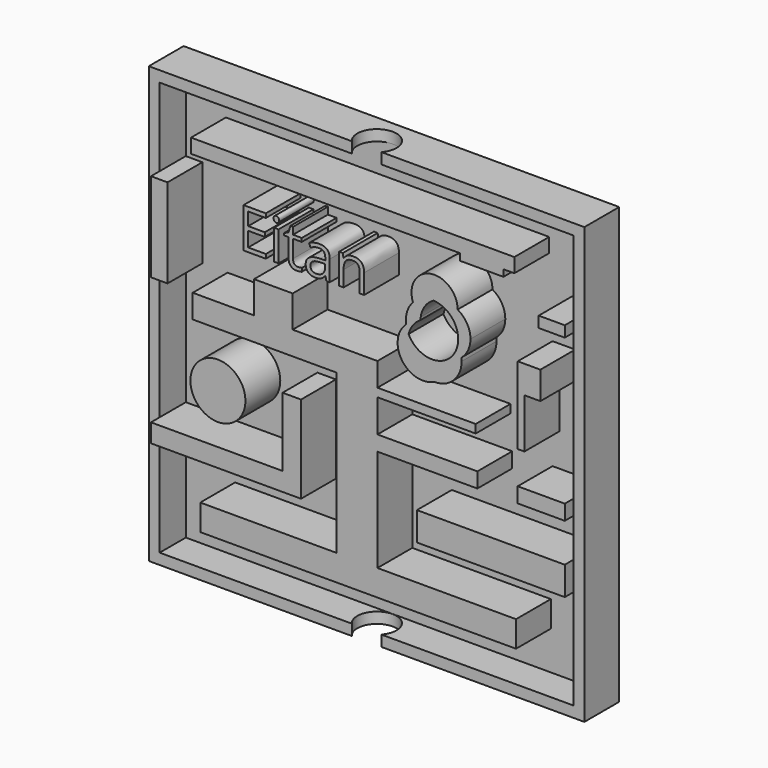
from build123d import *

# Parameters (mm, degrees)
F0_W         = 100
F0_H         = 100
F1_DEPTH     = 10
F2_T         = -2.5
F4_D         = 9
F5_W         = 22.9406361468
F5_H         = 3.4700129181
F5_W_2       = 22.5550816394
F5_H_2       = 1.9277847605
F5_W_3       = 8.8678086177
F5_H_3       = 7.3255812749
F5_W_4       = 4.2411256582
F5_H_4       = 15.8078335226
F5_R         = 6.314782536
F5_W_5       = 10.0244823843
F5_H_5       = 1.5422254801
F5_W_6       = 3.8039235713
F5_H_6       = 20.4345164821
F5_W_7       = 33.940872593
F5_H_7       = 6.5544676036
F5_W_8       = 10.8074559329
F5_W_9       = 1.5422254801
F5_H_8       = 17.7356194472
F5_W_10      = 5.9879957197
F5_H_9       = 2.5061201304
F5_TEXT_SIZE = 12.8518971097
F6_DEPTH     = 10
F7_W         = 3.6627911031
F7_H         = 6.3616903499
F8_DEPTH     = 10


# Not quite as in the source:
# - Text() gives the source's letters only with a copy of the font that has no kerning and outlines rounded to 1/6400 em; it was checked with that copy


with BuildPart() as f1:
    # F0 (on Front) → F1 (new body)
    with BuildSketch(Plane.XZ):
        with Locations((0.3209233341, -0.195864588)):
            Rectangle(F0_W, F0_H)
    extrude(amount=F1_DEPTH)

    # F2
    f2_openings = [f1.faces().sort_by_distance(p)[0] for p in [
        (0.320923, -10, -0.195865),
    ]]
    offset(amount=F2_T, openings=f2_openings)

    # F4 (through all)
    with Locations(Plane(origin=(0, 0, -50.195864588), x_dir=(1, 0, 0), z_dir=(0, 0, -1))):
        with Locations((0.3209233341, 7.0364135318)):
            Hole(F4_D / 2)

    # F5 (on face) → F6 (join)
    with BuildSketch(Plane.XZ.offset(2.5)):
        Polygon((-4.6266834252, -32.8687280416), (-35.8567945659, -32.8687280416), (-35.8567945659, -38.8448610902), (36.627907306, -38.8448610902), (36.627907306, -32.8687280416), (4.8194616102, -32.8687280416), align=None)
        Polygon((-4.6266834252, 0), (-4.6266834252, -32.8687280416), (4.8194616102, -32.8687280416), (4.8194616102, -10.5064269155), (4.8194616102, -9.3497559428), (4.8194616102, -5.8797430247), (4.8194616102, 0), align=None)
        Polygon((-4.6266834252, 3.5664017778), (-4.6266834252, 0), (4.8194616102, 0), (4.8194616102, 1.6386170173), (4.8194616102, 3.5664017778), align=None)
        Polygon((-4.8194616102, 3.5664017778), (-4.6266834252, 3.5664017778), (4.8194616102, 3.5664017778), (4.8194616102, 8.9641986415), (-4.8194616102, 8.9641986415), align=None)
        with Locations((16.2897796836, -7.6147494838)):
            Rectangle(F5_W, F5_H)
        with Locations((16.0970024299, 2.6025093975)):
            Rectangle(F5_W_2, F5_H_2)
        Polygon((-37.5918000937, 3.5664017778), (-4.8194616102, 3.5664017778), (-4.8194616102, 8.9641986415), (-14.6511634812, 8.9641986415), (-23.5189720988, 8.9641986415), (-37.5918000937, 8.9641986415), align=None)
        with Locations((-19.08506779, 12.6269892789)):
            Rectangle(F5_W_3, F5_H_3)
        Polygon((-47.1790766659, -20.3381273896), (-47.1790766659, -24.5792549103), (-12.7233788371, -24.5792549103), (-12.7233788371, -20.3381273896), (-16.9645044953, -20.3381273896), align=None)
        with Locations((-14.8439416662, -12.4342106283)):
            Rectangle(F5_W_4, F5_H_4)
        with Locations((-31.8084470928, -8.9641986415)):
            Circle(F5_R)
        Polygon((36.2423509359, 40.1943102479), (-37.9773564637, 40.1943102479), (-37.9773564637, 36.9170755148), (23.7117502838, 36.9170755148), (33.7362326682, 36.9170755148), (36.2423509359, 36.9170755148), align=None)
        with Locations((28.723991476, 36.1459627748)):
            Rectangle(F5_W_5, F5_H_5)
        with Locations((-45.2771148802, 19.1814568825)):
            Rectangle(F5_W_6, F5_H_6)
        with Locations((30.8504870376, -21.4947992936)):
            Rectangle(F5_W_7, F5_H_7)
        with Locations((42.4171953677, -7.6147494838)):
            Rectangle(F5_W_8, F5_H)
        with Locations((37.7845801413, 10.5064267409)):
            Rectangle(F5_W_9, F5_H_8)
        with BuildLine():
            ThreePointArc((24.0965098275, 15.9287748091), (25.6230664604, 17.9026526091), (26.1662343132, 20.3381273896))
            ThreePointArc((26.1662343132, 20.3381273896), (25.3756261323, 23.2429549658), (23.2219077195, 25.3464238964))
            ThreePointArc((23.2219077195, 25.3464238964), (23.0203095573, 23.9034058554), (22.4329388751, 22.5700122273))
            ThreePointArc((22.4329388751, 22.5700122273), (23.1192244348, 21.0371813988), (23.3541124158, 19.3742364645))
            ThreePointArc((23.3541124158, 19.3742364645), (23.3320620315, 18.860138238), (23.2660728424, 18.3498161507))
            ThreePointArc((23.2660728424, 18.3498161507), (23.807721157, 17.1826619431), (24.0965098275, 15.9287748091))
        make_face()
        with BuildLine():
            ThreePointArc((22.4329388751, 22.5700122273), (23.0203095573, 23.9034058554), (23.2219077195, 25.3464238964))
            ThreePointArc((23.2219077195, 25.3464238964), (20.4576770002, 26.0697974998), (17.6876908593, 25.3687856468))
            ThreePointArc((17.6876908593, 25.3687856468), (20.4002676099, 24.5457800283), (22.4329388751, 22.5700122273))
        make_face()
        with BuildLine():
            ThreePointArc((17.6876908593, 25.3687856468), (20.4576770002, 26.0697974998), (23.2219077195, 25.3464238964))
            ThreePointArc((23.2219077195, 25.3464238964), (23.2219088213, 25.3483957733), (23.2219091886, 25.3503676504))
            ThreePointArc((23.2219091886, 25.3503676504), (16.9805742217, 30.5583349113), (12.9743027111, 23.4853600249))
            ThreePointArc((12.9743027111, 23.4853600249), (15.1221825024, 24.9496433873), (17.6876908593, 25.3687856468))
        make_face()
        with BuildLine():
            ThreePointArc((24.1427720601, 15.1731938678), (24.131195683, 15.5516918047), (24.0965098275, 15.9287748091))
            ThreePointArc((24.0965098275, 15.9287748091), (22.6640607272, 15.0578134565), (21.0408778609, 14.6385742819))
            ThreePointArc((21.0408778609, 14.6385742819), (21.0187106408, 14.6213809917), (20.9964633286, 14.6042914634))
            ThreePointArc((20.9964633286, 14.6042914634), (21.0087530768, 14.3869085479), (21.0128515959, 14.1692170873))
            ThreePointArc((21.0128515959, 14.1692170873), (20.1405121578, 11.1148564843), (17.7866546853, 8.9819125591))
            ThreePointArc((17.7866546853, 8.9819125591), (22.2708562336, 10.7366357332), (24.1427720601, 15.1731938678))
        make_face()
        with BuildLine():
            ThreePointArc((21.0408778609, 14.6385742819), (22.6640607272, 15.0578134565), (24.0965098275, 15.9287748091))
            ThreePointArc((24.0965098275, 15.9287748091), (23.807721157, 17.1826619431), (23.2660728424, 18.3498161507))
            ThreePointArc((23.2660728424, 18.3498161507), (22.4994415144, 16.2867600244), (21.0408778609, 14.6385742819))
        make_face()
        with BuildLine():
            ThreePointArc((14.7554455633, 21.1131896721), (15.7147223697, 23.5902210791), (17.6876908593, 25.3687856468))
            ThreePointArc((17.6876908593, 25.3687856468), (15.1221825024, 24.9496433873), (12.9743027111, 23.4853600249))
            ThreePointArc((12.9743027111, 23.4853600249), (13.6953110526, 22.1719584963), (14.7554455633, 21.1131896721))
        make_face()
        with BuildLine():
            ThreePointArc((14.7038566182, 20.4481522521), (14.7199685728, 20.781422064), (14.7554455633, 21.1131896721))
            ThreePointArc((14.7554455633, 21.1131896721), (13.6953110526, 22.1719584963), (12.9743027111, 23.4853600249))
            ThreePointArc((12.9743027111, 23.4853600249), (11.6230003713, 21.1768372017), (11.4084636735, 18.5105158325))
            ThreePointArc((11.4084636735, 18.5105158325), (12.5307742708, 19.2842995338), (13.8030257235, 19.7738897037))
            ThreePointArc((13.8030257235, 19.7738897037), (14.2380969143, 20.1315212718), (14.7038566182, 20.4481522521))
        make_face()
        with BuildLine():
            ThreePointArc((21.0128515959, 14.1692170873), (21.0087530768, 14.3869085479), (20.9964633286, 14.6042914634))
            ThreePointArc((20.9964633286, 14.6042914634), (15.9717620607, 13.5305304551), (11.9564739707, 16.7364698008))
            ThreePointArc((11.9564739707, 16.7364698008), (12.9989922821, 11.4513179657), (17.7866546853, 8.9819125591))
            ThreePointArc((17.7866546853, 8.9819125591), (20.1405121578, 11.1148564843), (21.0128515959, 14.1692170873))
        make_face()
        with BuildLine():
            ThreePointArc((11.4084636735, 18.5105158325), (10.4234688224, 10.9521902624), (17.7866546853, 8.9819125591))
            ThreePointArc((17.7866546853, 8.9819125591), (12.9989922821, 11.4513179657), (11.9564739707, 16.7364698008))
            ThreePointArc((11.9564739707, 16.7364698008), (11.6134757189, 17.6021805562), (11.4084636735, 18.5105158325))
        make_face()
        with BuildLine():
            ThreePointArc((13.8030257235, 19.7738897037), (12.5307742708, 19.2842995338), (11.4084636735, 18.5105158325))
            ThreePointArc((11.4084636735, 18.5105158325), (11.6134757189, 17.6021805562), (11.9564739707, 16.7364698008))
            ThreePointArc((11.9564739707, 16.7364698008), (12.6571553581, 18.3905025779), (13.8030257235, 19.7738897037))
        make_face()
        with Locations((44.8269254743, 28.916769661)):
            Rectangle(F5_W_10, F5_H_9)
        with Locations((-27.181763202, 21.3020201772)):
            Text('Eitan', F5_TEXT_SIZE, font='Open Sans', text_align=(TextAlign.LEFT, TextAlign.BOTTOM))
    extrude(amount=F6_DEPTH)

    # F7 (on face) → F8 (join)
    with BuildSketch(Plane.XZ.offset(2.5)):
        with Locations((40.3870884329, 16.1933912896)):
            Rectangle(F7_W, F7_H)
    extrude(amount=F8_DEPTH)


solid = f1.part
